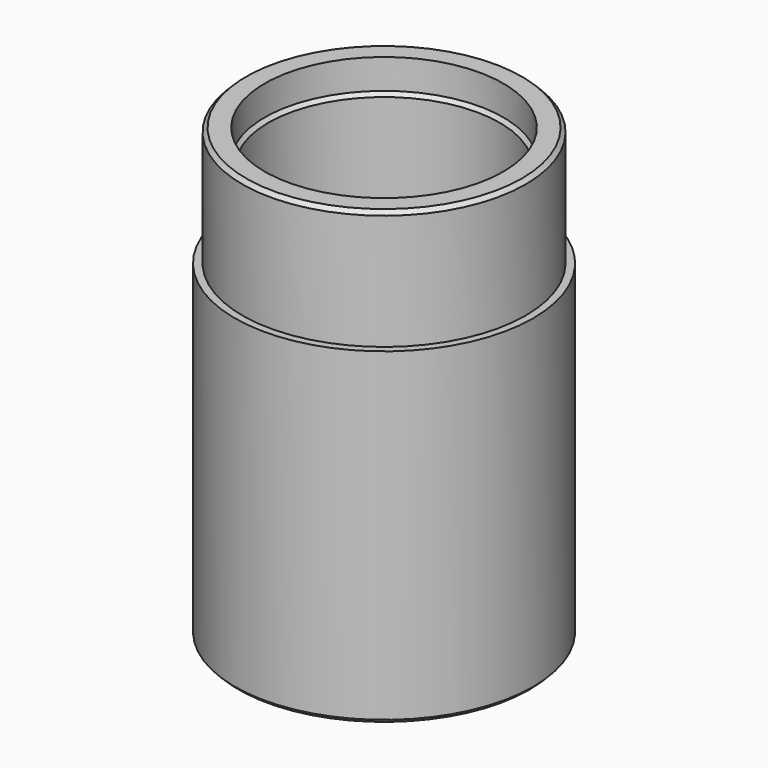
from build123d import *

# Parameters (mm, degrees)
F0_R     = 30.1625
F1_DEPTH = 6.35
F2_R     = 31.75
F3_DEPTH = 69.85
F4_R     = 30.1625
F5_DEPTH = 12.7
F6_R     = 24.638
F7_DEPTH = 95.251
F8_R     = 25.4
F9_DEPTH = 6.35
F10_SIZE = 0.76199
F11_SIZE = 1.5875
F12_SIZE = 0.8255


# Not quite as in the source:
# - a fillet or chamfer is up to 0.001 mm smaller than in the source, because OpenCascade refuses the exact size


with BuildPart() as f1:
    # F0 (on Top) → F1 (new body, symmetric)
    with BuildSketch(Plane.XY):
        Circle(F0_R)
    extrude(amount=F1_DEPTH, both=True)

    # F2 (on face) → F3 (join)
    with BuildSketch(Plane(origin=(0, 0, -6.35), x_dir=(1, 0, 0), z_dir=(0, 0, -1))):
        Circle(F2_R)
    extrude(amount=F3_DEPTH)

    # F4 (on face) → F5 (join)
    with BuildSketch(Plane.XY.offset(6.35)):
        Circle(F4_R)
    extrude(amount=F5_DEPTH)

    # F6 (on face) → F7 (cut, through all)
    with BuildSketch(Plane.XY.offset(19.05)):
        Circle(F6_R)
    extrude(amount=-F7_DEPTH, mode=Mode.SUBTRACT)

    # F8 (on face) → F9 (cut)
    with BuildSketch(Plane.XY.offset(19.05)):
        Circle(F8_R)
    extrude(amount=-F9_DEPTH, mode=Mode.SUBTRACT)

    # F10 (size 0.762 in the source; OpenCascade refuses exactly that, so slightly less here)
    f10_edges = [f1.edges().sort_by_distance(p)[0] for p in [
        (-24.638, 0, 12.7),
    ]]
    chamfer(f10_edges, length=F10_SIZE)

    # F11
    f11_edges = [f1.edges().sort_by_distance(p)[0] for p in [
        (-24.638, 0, -76.2),
    ]]
    chamfer(f11_edges, length=F11_SIZE)

    # F12
    f12_edges = [f1.edges().sort_by_distance(p)[0] for p in [
        (-31.75, 0, -76.2),
        (-30.1625, 0, 19.05),
    ]]
    chamfer(f12_edges, length=F12_SIZE)


solid = f1.part
